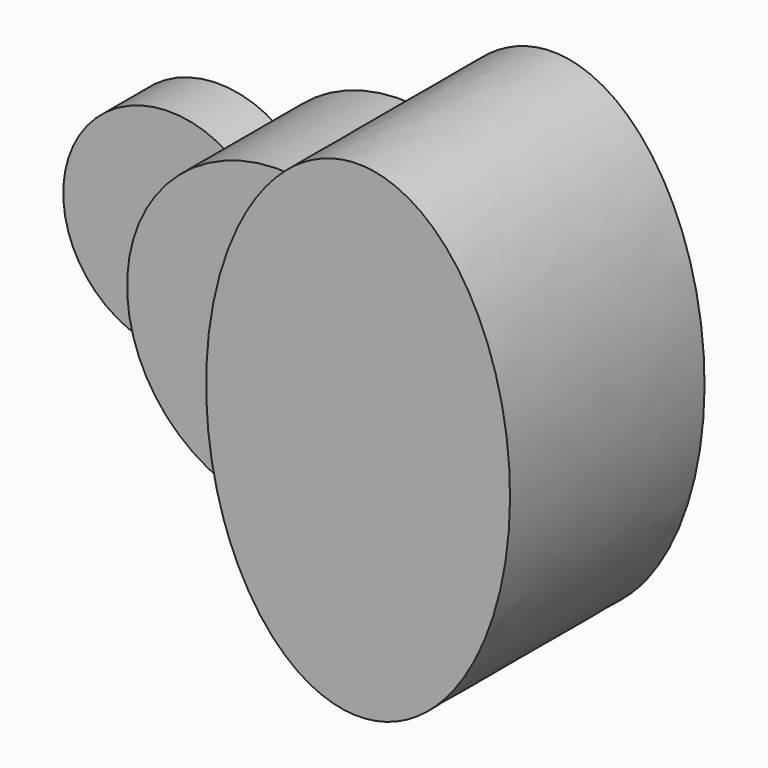
from build123d import *

# Parameters (mm, degrees)
F1_DEPTH = 25.4
F2_DEPTH = 63.5
F3_DEPTH = 101.6


with BuildPart() as f1:
    # F0 (on Front) → F1 (new body)
    with BuildSketch(Plane.XZ):
        with BuildLine():
            ThreePointArc((-51.59375, -37.018036), (-63.5, 0), (-51.59375, 37.018036))
            ThreePointArc((-51.59375, 37.018036), (-120.65, 0), (-51.59375, -37.018036))
        make_face()
    extrude(amount=F1_DEPTH)

    # F0 (on Front) → F2 (join)
    with BuildSketch(Plane.XZ):
        with BuildLine():
            ThreePointArc((-51.59375, -37.018036), (-37.023793, -21.000651), (-31.75, 0))
            ThreePointArc((-31.75, 0), (-37.023793, 21.000651), (-51.59375, 37.018036))
            ThreePointArc((-51.59375, 37.018036), (-63.5, 0), (-51.59375, -37.018036))
        make_face()
        with BuildLine():
            ThreePointArc((-51.59375, 37.018036), (-37.023793, 21.000651), (-31.75, 0))
            ThreePointArc((-31.75, 0), (-37.023793, -21.000651), (-51.59375, -37.018036))
            ThreePointArc((-51.59375, -37.018036), (-22.912811, -59.222066), (13.243966, -62.103521))
            add(Edge.make_bspline(
                [(0, 0), (0, -34.66694), (13.243966, -62.103521)],
                knots=[4.712389, 4.712389, 4.712389, 5.370034, 5.370034, 5.370034], degree=2, weights=[1, 0.946423, 1]))
            add(Edge.make_bspline(
                [(13.243966, 62.103521), (0, 34.66694), (0, 0)],
                knots=[4.054743, 4.054743, 4.054743, 4.712389, 4.712389, 4.712389], degree=2, weights=[1, 0.946423, 1]))
            ThreePointArc((13.243966, 62.103521), (-22.912811, 59.222066), (-51.59375, 37.018036))
        make_face()
    extrude(amount=F2_DEPTH)

    # F0 (on Front) → F3 (join)
    with BuildSketch(Plane.XZ):
        with BuildLine():
            ThreePointArc((63.5, 0), (49.36214, 39.945326), (13.243966, 62.103521))
            add(Edge.make_bspline(
                [(13.243966, 62.103521), (0, 34.66694), (0, 0)],
                knots=[4.054743, 4.054743, 4.054743, 4.712389, 4.712389, 4.712389], degree=2, weights=[1, 0.946423, 1]))
            add(Edge.make_bspline(
                [(0, 0), (0, -34.66694), (13.243966, -62.103521)],
                knots=[4.712389, 4.712389, 4.712389, 5.370034, 5.370034, 5.370034], degree=2, weights=[1, 0.946423, 1]))
            ThreePointArc((13.243966, -62.103521), (49.36214, -39.945326), (63.5, 0))
        make_face()
        with BuildLine():
            add(Edge.make_bspline(
                [(13.243966, -62.103521), (127, -297.763807), (127, 0), (127, 297.763807), (13.243966, 62.103521)],
                knots=[5.370034, 5.370034, 5.370034, 7.853982, 7.853982, 10.337929, 10.337929, 10.337929], degree=2, weights=[1, 0.322929, 1, 0.322929, 1]))
            ThreePointArc((13.243966, 62.103521), (49.36214, 39.945326), (63.5, 0))
            ThreePointArc((63.5, 0), (49.36214, -39.945326), (13.243966, -62.103521))
        make_face()
    extrude(amount=F3_DEPTH)


solid = f1.part
